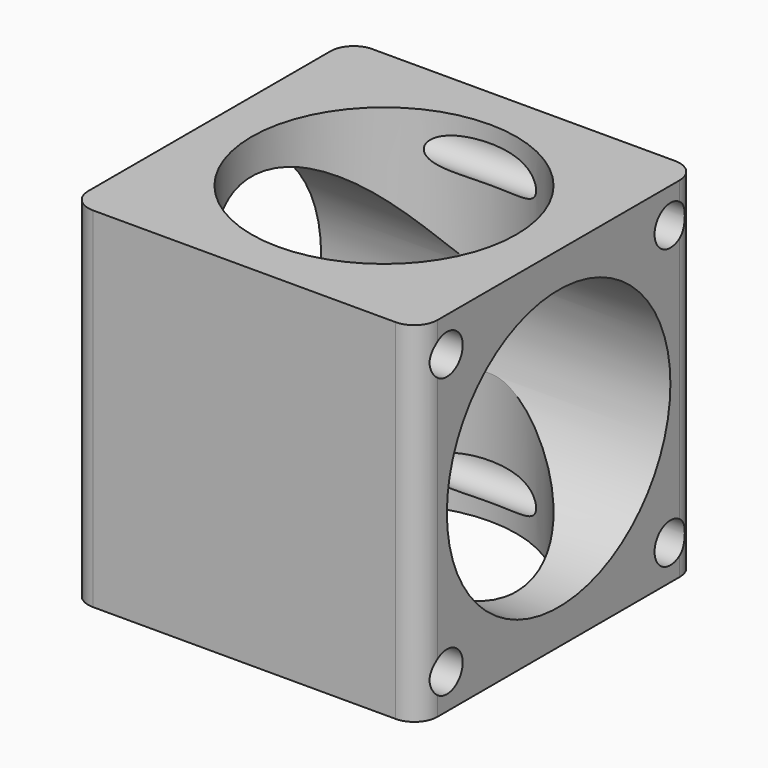
from build123d import *

# Parameters (mm, degrees)
F0_W        = 30
F0_H        = 30
F0_R        = 11.375
F1_DEPTH    = 30
F3_D        = 3.4
F4_T1_DEPTH = 40
F2_R        = 12
F5_DEPTH    = 30.0010001


# Not quite as in the source:
# - a fillet or chamfer that OpenCascade refuses, or shapes differently, is made with other operations: its cross-section is extruded or revolved along the edge and cut away or added


with BuildPart() as f1:
    # F0 (on Top) → F1 (new body)
    with BuildSketch(Plane.XY):
        Rectangle(F0_W, F0_H)
        Circle(F0_R, mode=Mode.SUBTRACT)
    extrude(amount=F1_DEPTH)

    # F3 (through all)
    with Locations(Plane(origin=(-15, 0, 0), x_dir=(0, -1, 0), z_dir=(-1, 0, 0))):
        with Locations((-12, 27), (12, 27), (12, 3), (-12, 3)):
            Hole(F3_D / 2)

    # F4: fillet of radius 2 on 4 edges, made by hand

    # F4_s2 → F4_t1 (cut)
    with BuildSketch(Plane.XY.offset(-5)):
        with BuildLine():
            ThreePointArc((15, 13), (14.4142135624, 14.4142135624), (13, 15))
            Line((13, 15), (15, 15))
            Line((15, 15), (15, 13))
        make_face()
        with BuildLine():
            ThreePointArc((-15, 13), (-14.4142135624, 14.4142135624), (-13, 15))
            Line((-13, 15), (-15, 15))
            Line((-15, 15), (-15, 13))
        make_face()
        with BuildLine():
            ThreePointArc((-13, -15), (-14.4142135624, -14.4142135624), (-15, -13))
            Line((-15, -13), (-15, -15))
            Line((-15, -15), (-13, -15))
        make_face()
        with BuildLine():
            ThreePointArc((13, -15), (14.4142135624, -14.4142135624), (15, -13))
            Line((15, -13), (15, -15))
            Line((15, -15), (13, -15))
        make_face()
    extrude(amount=F4_T1_DEPTH, mode=Mode.SUBTRACT)

    # F2 (on face) → F5 (cut, through all)
    with BuildSketch(Plane(origin=(-15, 0, 0), x_dir=(0, -1, 0), z_dir=(-1, 0, 0))):
        with Locations((0, 15)):
            Circle(F2_R)
    extrude(amount=-F5_DEPTH, mode=Mode.SUBTRACT)


solid = f1.part
